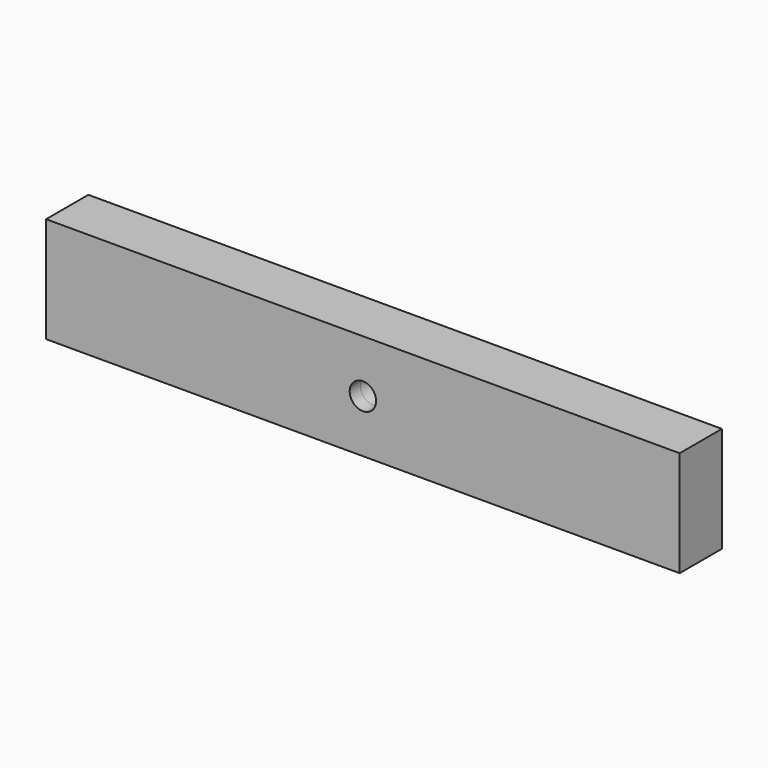
from build123d import *

# Parameters (mm, degrees)
F0_W     = 304.8
F0_H     = 50.8
F0_R     = 6.35
F1_DEPTH = 19.05


# Not quite as in the source:
# - a pattern or mirror of a feature is missing from the dataset's text; its kind, count and spacing are read off the source's solid


with BuildPart() as f1:
    # F0 (on Front) → F1 (new body)
    with BuildSketch(Plane.XZ):
        Rectangle(F0_W, F0_H)
        Circle(F0_R, mode=Mode.SUBTRACT)
    extrude(amount=F1_DEPTH)

    # F1_copies: F1 across plane


with BuildPart() as f1_1:
    add(f1.part)
    add(f1.part.mirror(Plane(origin=(0, -12.7, 0), x_dir=(0, 0, -1), z_dir=(0, -1, 0))))


solid = f1_1.part
